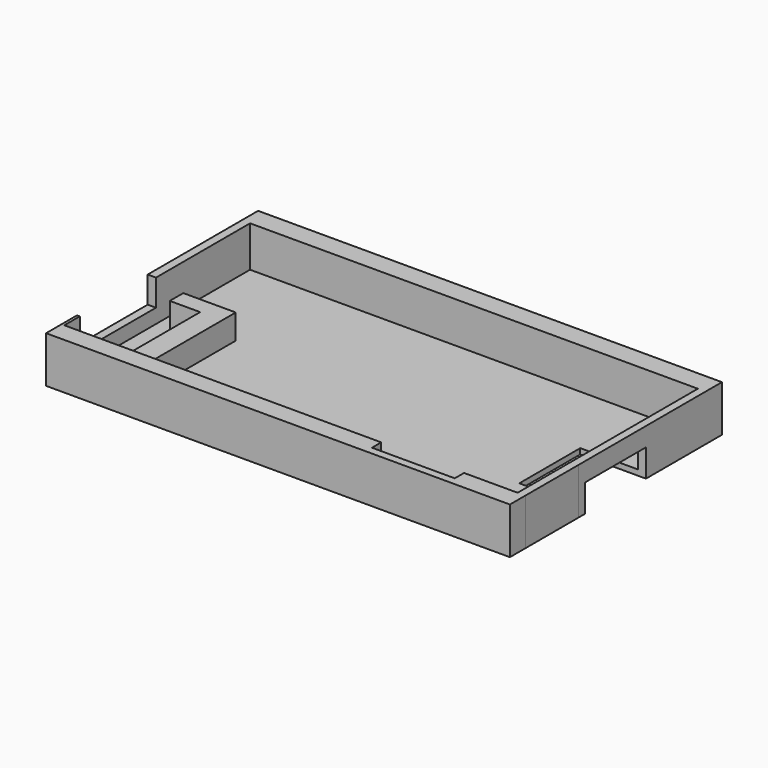
from build123d import *

# Parameters (mm, degrees)
F0_W     = 4
F0_H     = 16
F1_DEPTH = 1
F0_W_2   = 1.4000003636
F0_H_2   = 11.8
F0_H_3   = 2
F2_DEPTH = 7.4
F3_DEPTH = 2.6
F4_DEPTH = 4.5
F5_DEPTH = 4


# Not quite as in the source:
# - ends of sketch curves that miss each other by under 0.0002 mm in the source are joined
# - a feature names something its author has since deleted; it is built from what else it names


with BuildPart() as f1:
    # F0 (on Top) → F1 (new body)
    with BuildSketch(Plane.XY):
        Polygon((-46.6793118417, -34.5732776225), (-46.6793118417, -35.6732776225), (9.7206891477, -35.6732776225), (9.7206891477, -37.6732772589), (19.7206891477, -37.6732772589), (19.7206891477, -35.5732776225), (29.4207941621, -35.5732776225), (29.4207941621, -34.5732776225), (31.9206877947, -34.5732776225), (31.9206877947, -26.0732776225), (29.4206877947, -26.0732776225), (29.4206877947, -24.5732776225), (21.4206877947, -24.5732776225), (21.4206877947, -12.7732776225), (21.4206877947, -10.7732776225), (29.4206877947, -10.7732776225), (29.4206877947, 0.2267237306), (-46.6793118417, 0.2267237306), (-46.6793118417, -15.5122037977), (-37.1793118417, -15.5122037977), (-37.1793118417, -18.5732776225), (-37.1793118417, -34.5732776225), (-41.1793118417, -34.5732776225), (-41.1793118417, -18.5732776225), (-46.6793118417, -18.5732776225), (-49.1793118417, -18.5732776225), (-49.1793118417, -34.5732776225), align=None)
        Polygon((-49.1793118417, 2.7267237306), (-49.1793118417, -18.5732776225), (-46.6793118417, -18.5732776225), (-46.6793118417, -15.5122037977), (-46.6793118417, 0.2267237306), (29.4206877947, 0.2267237306), (29.4206877947, -10.7732776225), (31.9206877947, -10.7732776225), (31.9206877947, 2.7267237306), align=None)
        Polygon((-50.6793118417, -1.5732776225), (-50.6793118417, -18.5732776225), (-49.1793118417, -18.5732776225), (-49.1793118417, 2.7267237306), (31.9206877947, 2.7267237306), (31.9206877947, -10.7732776225), (33.3206881583, -10.7732776225), (33.3206881583, 6.4267223775), (30.3206881583, 6.4267223775), (-50.6793118417, 6.4267223775), align=None)
        Polygon((-46.6793118417, -35.6732776225), (-46.6793118417, -38.0732776225), (7.2206891477, -38.0732776225), (7.2206891477, -40.1732772589), (22.2206891477, -40.1732772589), (22.2206891477, -38.0732776225), (29.4207941621, -38.0732776225), (31.9206877947, -38.0732776225), (31.9206877947, -34.5732776225), (29.4207941621, -34.5732776225), (29.4207941621, -35.5732776225), (19.7206891477, -35.5732776225), (19.7206891477, -37.6732772589), (9.7206891477, -37.6732772589), (9.7206891477, -35.6732776225), align=None)
        Polygon((-50.6793118417, -38.0732776225), (-50.6793118417, -41.5732776225), (30.3206881583, -41.5732776225), (33.3206881583, -41.5732776225), (33.3206349746, -38.0732776225), (31.9206877947, -38.0732776225), (29.4207941621, -38.0732776225), (22.2206891477, -38.0732776225), (22.2206891477, -40.1732772589), (7.2206891477, -40.1732772589), (7.2206891477, -38.0732776225), (-46.6793118417, -38.0732776225), (-50.1793118417, -38.0732776225), align=None)
        Polygon((31.9206877947, -26.0732776225), (33.3206881583, -26.0732776225), (33.3206881583, -24.5732776225), (31.9206877947, -24.5732776225), (31.9206877947, -25.7732776225), align=None)
        Polygon((33.3205817909, -34.5732776225), (33.3206349746, -38.0732776225), (33.3206881583, -26.0732776225), (31.9206877947, -26.0732776225), (31.9206877947, -34.5732776225), align=None)
        Polygon((31.9206877947, -38.0732776225), (33.3206349746, -38.0732776225), (33.3205817909, -34.5732776225), (31.9206877947, -34.5732776225), align=None)
        Polygon((-50.6793118417, -18.5732776225), (-50.6793118417, -34.5732776225), (-50.1793118417, -34.5732776225), (-49.1793118417, -34.5732776225), (-49.1793118417, -18.5732776225), align=None)
        Polygon((-50.1793118417, -34.5732776225), (-50.1793118417, -38.0732776225), (-46.6793118417, -38.0732776225), (-46.6793118417, -35.6732776225), (-46.6793118417, -34.5732776225), (-49.1793118417, -34.5732776225), align=None)
        Polygon((-50.6793118417, -35.5732776225), (-50.6793118417, -38.0732776225), (-50.1793118417, -38.0732776225), (-50.1793118417, -34.5732776225), (-50.6793118417, -34.5732776225), align=None)
        with Locations((-39.1793118417, -26.5732776225)):
            Rectangle(F0_W, F0_H)
        Polygon((-46.6793118417, -15.5122037977), (-46.6793118417, -18.5732776225), (-41.1793118417, -18.5732776225), (-37.1793118417, -18.5732776225), (-37.1793118417, -15.5122037977), align=None)
        Polygon((29.4206877947, -26.0732776225), (31.9206877947, -26.0732776225), (31.9206877947, -25.7732776225), (31.9206877947, -24.5732776225), (29.4206877947, -24.5732776225), align=None)
    extrude(amount=-F1_DEPTH)

    # F0 (on Top) → F2 (join)
    with BuildSketch(Plane.XY):
        Polygon((-50.6793118417, -38.0732776225), (-50.6793118417, -41.5732776225), (30.3206881583, -41.5732776225), (33.3206881583, -41.5732776225), (33.3206349746, -38.0732776225), (31.9206877947, -38.0732776225), (29.4207941621, -38.0732776225), (22.2206891477, -38.0732776225), (22.2206891477, -40.1732772589), (7.2206891477, -40.1732772589), (7.2206891477, -38.0732776225), (-46.6793118417, -38.0732776225), (-50.1793118417, -38.0732776225), align=None)
        Polygon((-50.6793118417, -1.5732776225), (-50.6793118417, -18.5732776225), (-49.1793118417, -18.5732776225), (-49.1793118417, 2.7267237306), (31.9206877947, 2.7267237306), (31.9206877947, -10.7732776225), (33.3206881583, -10.7732776225), (33.3206881583, 6.4267223775), (30.3206881583, 6.4267223775), (-50.6793118417, 6.4267223775), align=None)
        Polygon((31.9206877947, -26.0732776225), (33.3206881583, -26.0732776225), (33.3206881583, -24.5732776225), (31.9206877947, -24.5732776225), (31.9206877947, -25.7732776225), align=None)
        Polygon((33.3205817909, -34.5732776225), (33.3206349746, -38.0732776225), (33.3206881583, -26.0732776225), (31.9206877947, -26.0732776225), (31.9206877947, -34.5732776225), align=None)
        Polygon((31.9206877947, -38.0732776225), (33.3206349746, -38.0732776225), (33.3205817909, -34.5732776225), (31.9206877947, -34.5732776225), align=None)
        Polygon((-50.6793118417, -35.5732776225), (-50.6793118417, -38.0732776225), (-50.1793118417, -38.0732776225), (-50.1793118417, -34.5732776225), (-50.6793118417, -34.5732776225), align=None)
        with Locations((32.6206879765, -18.6732776225)):
            Rectangle(F0_W_2, F0_H_2)
        with Locations((32.6206879765, -11.7732776225)):
            Rectangle(F0_W_2, F0_H_3)
    extrude(amount=F2_DEPTH)

    # F0 (on Top) → F3 (join)
    with BuildSketch(Plane.XY):
        Polygon((-50.6793118417, -18.5732776225), (-50.6793118417, -34.5732776225), (-50.1793118417, -34.5732776225), (-49.1793118417, -34.5732776225), (-49.1793118417, -18.5732776225), align=None)
    extrude(amount=F3_DEPTH)

    # F0 (on Top) → F4 (join)
    with BuildSketch(Plane.XY):
        with Locations((-39.1793118417, -26.5732776225)):
            Rectangle(F0_W, F0_H)
        Polygon((-46.6793118417, -15.5122037977), (-46.6793118417, -18.5732776225), (-41.1793118417, -18.5732776225), (-37.1793118417, -18.5732776225), (-37.1793118417, -15.5122037977), align=None)
    extrude(amount=F4_DEPTH)

    # F0 (on Top) → F5 (cut)
    with BuildSketch(Plane.XY):
        with Locations((32.6206879765, -18.6732776225)):
            Rectangle(F0_W_2, F0_H_2)
        with Locations((32.6206879765, -11.7732776225)):
            Rectangle(F0_W_2, F0_H_3)
    extrude(amount=F5_DEPTH, mode=Mode.SUBTRACT)


solid = f1.part
